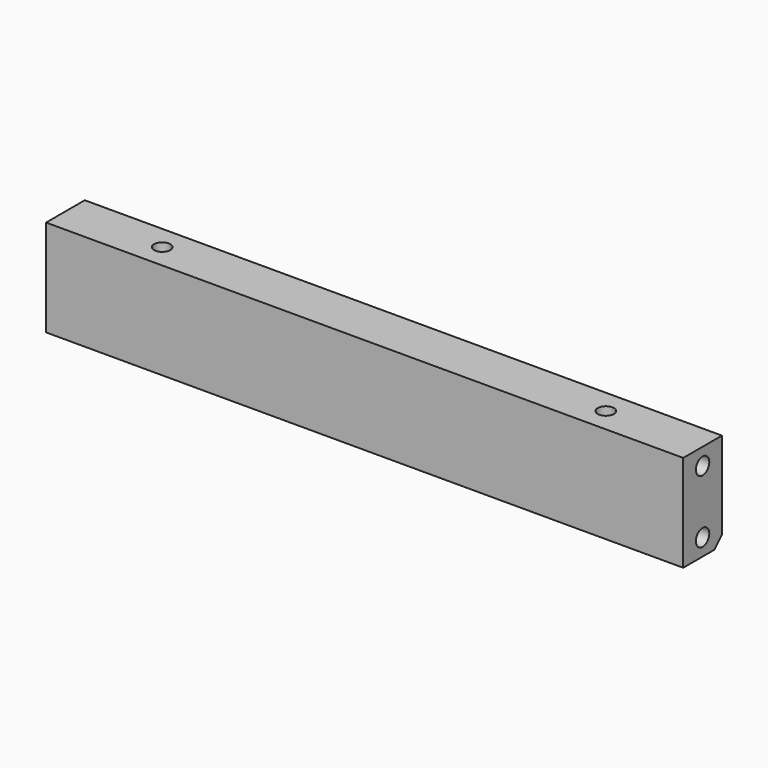
from build123d import *

# Parameters (mm, degrees)
F0_W           = 334.6
F0_H           = 25.4
F1_DEPTH       = 50.8
F4_D           = 8.8
F4_DEPTH       = 23.1302
F4_TIP         = 2.6437867237
F4_ON_F2_D     = 8.8
F4_ON_F2_DEPTH = 23.1302
F4_ON_F2_TIP   = 2.6437867237
F5_SIZE        = 5.08
F7_D           = 8.5


# Not quite as in the source:
# - a feature names something its author has since deleted; it is built from what else it names


with BuildPart() as f1:
    # F0 (on Top) → F1 (new body)
    with BuildSketch(Plane.XY):
        with Locations((164.5870582715, 12.7)):
            Rectangle(F0_W, F0_H)
    extrude(amount=F1_DEPTH)

    # F4
    with Locations(Plane(origin=(-2.7129417285, 0, 0), x_dir=(0, -1, 0), z_dir=(-1, 0, 0))):
        with Locations((-12.7, 41.91), (-12.7, 8.89)):
            Hole(F4_D / 2, depth=F4_DEPTH)
            with Locations((0, 0, -(F4_DEPTH + F4_TIP / 2))):  # 118° drill point
                Cone(0, F4_D / 2, F4_TIP, mode=Mode.SUBTRACT)

    # F4 on F2
    with Locations(Plane.YZ.offset(331.8870582715)):
        with Locations((12.7, 41.91), (12.7, 8.89)):
            Hole(F4_ON_F2_D / 2, depth=F4_ON_F2_DEPTH)
            with Locations((0, 0, -(F4_ON_F2_DEPTH + F4_ON_F2_TIP / 2))):  # 118° drill point
                Cone(0, F4_ON_F2_D / 2, F4_ON_F2_TIP, mode=Mode.SUBTRACT)

    # F5
    f5_edges = [f1.edges().sort_by_distance(p)[0] for p in [
        (164.587058, 25.4, 0),
    ]]
    chamfer(f5_edges, length=F5_SIZE)

    # F7 (through all)
    with Locations(Plane(origin=(0, 0, 0), x_dir=(1, 0, 0), z_dir=(0, 0, -1))):
        with Locations((48.0870582715, -12.7), (281.0870582715, -12.7)):
            Hole(F7_D / 2)


solid = f1.part
